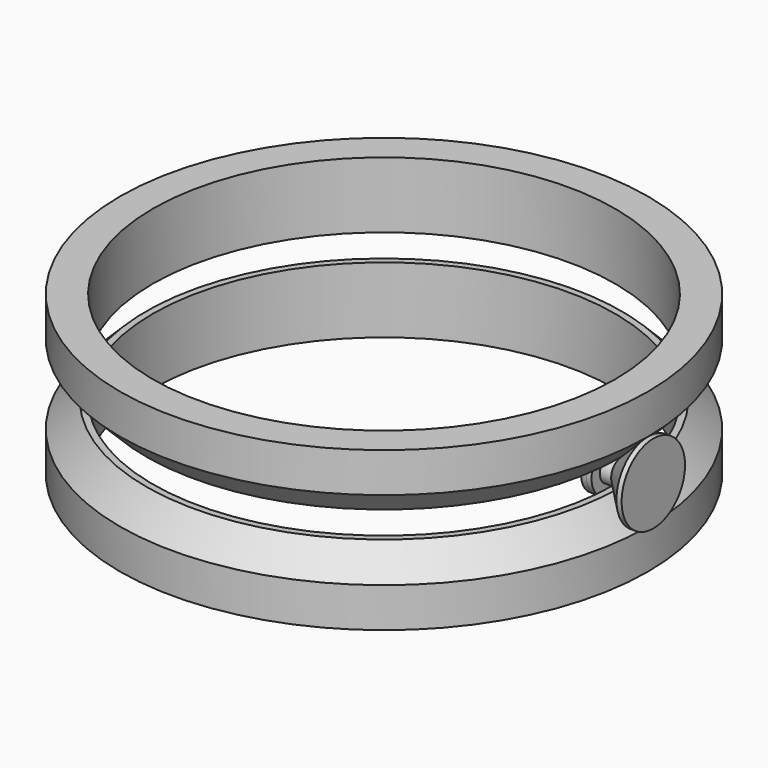
from build123d import *

# Parameters (mm, degrees)
F0_R      = 50.8
F0_R_2    = 44.45
F1_DEPTH  = 12.7
F2_SIZE   = 5.08
F4_R      = 7.62
F5_DEPTH  = 5.08
F6_SIZE   = 5.07999
F7_DEPTH  = 3.175
F10_R     = 4.54
F10_R_2   = 2.54
F11_DEPTH = 1
F12_DEPTH = 1
F13_DEPTH = 1


# Not quite as in the source:
# - a fillet or chamfer is up to 0.001 mm smaller than in the source, because OpenCascade refuses the exact size


with BuildPart() as f1:
    # F0 (on Top) → F1 (new body)
    with BuildSketch(Plane.XY):
        Circle(F0_R)
        Circle(F0_R_2, mode=Mode.SUBTRACT)
    extrude(amount=F1_DEPTH)

    # F2
    f2_edges = [f1.edges().sort_by_distance(p)[0] for p in [
        (-50.8, 0, 12.7),
    ]]
    chamfer(f2_edges, length=F2_SIZE)


with BuildPart() as f5:
    # F4 (on offset) → F5 (new body)
    with BuildSketch(Plane.YZ.offset(50.8)):
        with Locations((0, 15.24)):
            Circle(F4_R)
    extrude(amount=-F5_DEPTH)

    # F6 (size 5.08 in the source; OpenCascade refuses exactly that, so slightly less here)
    f6_edges = [f5.edges().sort_by_distance(p)[0] for p in [
        (45.72, -7.62, 15.24),
    ]]
    chamfer(f6_edges, length=F6_SIZE)

    # F7 (add): a face of the model
    f7_faces = [f5.faces().sort_by_distance(p)[0] for p in [
        (45.72, 0, 15.24),
    ]]
    extrude(f7_faces, amount=F7_DEPTH)

    # F10 (on face) → F11 (join)
    with BuildSketch(Plane(origin=(42.545, 0, 0), x_dir=(0, -1, 0), z_dir=(-1, 0, 0))):
        with Locations((0, 15.24)):
            Circle(F10_R)
        with Locations((0, 15.24)):
            Circle(F10_R_2, mode=Mode.SUBTRACT)
    extrude(amount=-F11_DEPTH)

    # F12 (add): a face of the model
    f12_faces = [f5.faces().sort_by_distance(p)[0] for p in [
        (42.545, 0, 15.24),
    ]]
    extrude(f12_faces, amount=F12_DEPTH)

    # F13 (add): a face of the model
    f13_faces = [f5.faces().sort_by_distance(p)[0] for p in [
        (50.8, 0, 15.24),
    ]]
    extrude(f13_faces, amount=F13_DEPTH)


with BuildPart() as f9_1:
    # F9: instance of F1
    add(f1.part.mirror(Plane.XY.offset(15.24)))


solid = Compound([f1.part, f5.part, f9_1.part])
